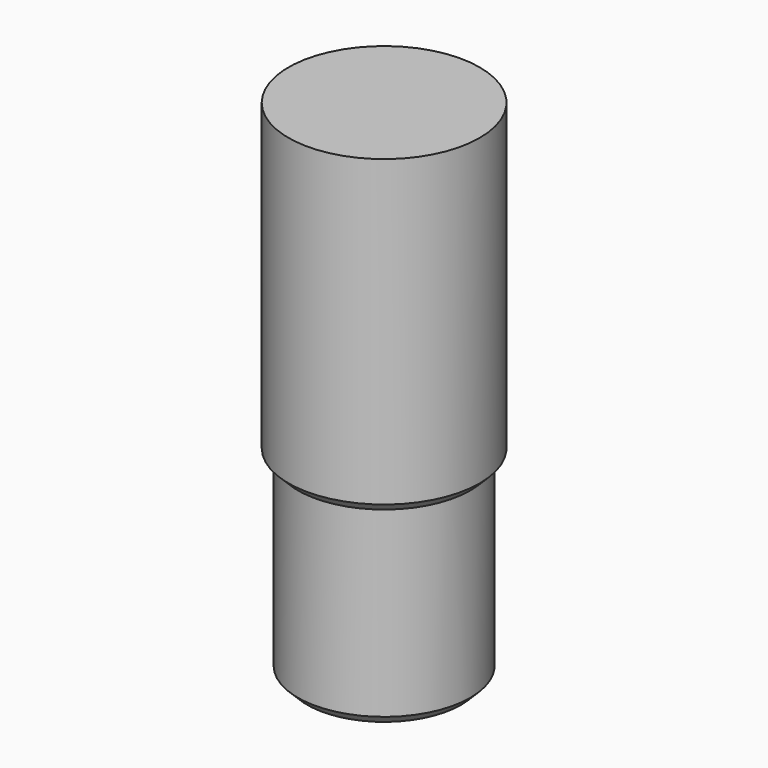
from build123d import *

# Parameters (mm, degrees)
F0_R        = 39.1254691666
F1_DEPTH    = 124.46
F2_R        = 35.3178604587
F3_DEPTH    = 82.296
F4_S5_R     = 39.1254691666
F4_T6_DEPTH = 57


# Not quite as in the source:
# - a fillet or chamfer that OpenCascade refuses, or shapes differently, is made with other operations: its cross-section is extruded or revolved along the edge and cut away or added
# - a feature of the source that left no trace in its solid (it failed there, or was rolled back) is left out


with BuildPart() as f1:
    # F0 (on Top) → F1 (new body)
    with BuildSketch(Plane.XY):
        Circle(F0_R)
    extrude(amount=F1_DEPTH)

    # F2 (on Top) → F3 (join)
    with BuildSketch(Plane.XY):
        Circle(F2_R)
    extrude(amount=-F3_DEPTH)

    # F4: chamfer of 3.81 on 3 edges, made by hand


with BuildPart() as f4_tool2:
    # F4_s3 → F4_t4 (revolve)
    with BuildSketch(Plane.XZ):
        Polygon((39.1278604587, 0), (35.3178604587, -3.81), (35.3178604587, 0), align=None)
    revolve(axis=Axis((0, 0, 0), (0, 0, 1)))

    # F4_s5 → F4_t6 (intersect, symmetric)
    with BuildSketch(Plane.XY.offset(-1.9)):
        Circle(F4_S5_R)
    extrude(amount=F4_T6_DEPTH, both=True, mode=Mode.INTERSECT)


with BuildPart() as f1_1:
    add(f1.part)

    # F4_t1: union F4_tool2
    add(f4_tool2.part)

    # F4_s7 → F4_t8 (revolve, cut)
    with BuildSketch(Plane.XZ):
        Polygon((35.3178604587, -78.486), (31.5078604587, -82.296), (35.3178604587, -82.296), align=None)
    revolve(axis=Axis((0, 0, -82.296), (0, 0, 1)), mode=Mode.SUBTRACT)


solid = f1_1.part
